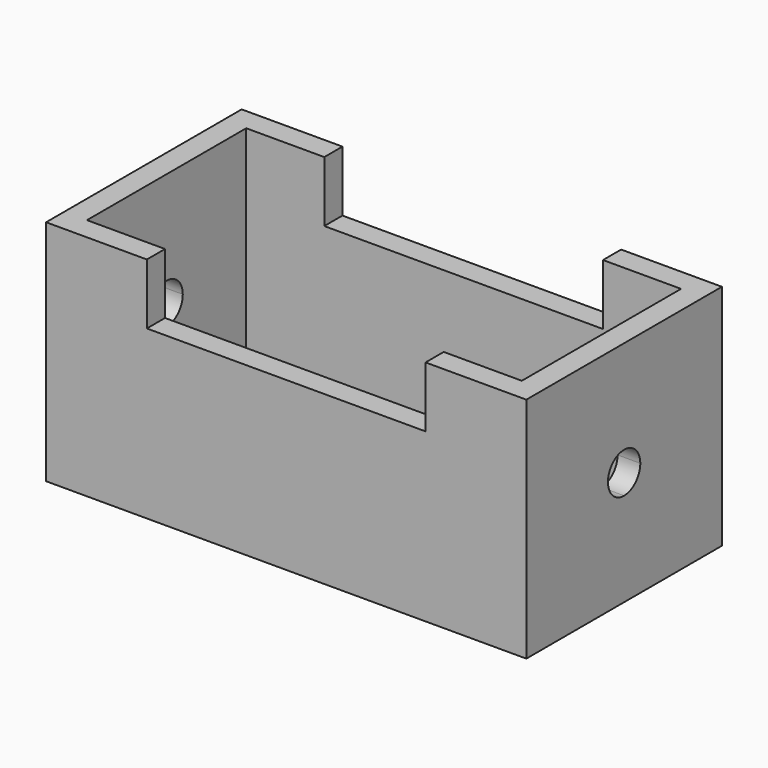
from build123d import *
from build123d import SkipClean  # not in build123d's __all__

# Parameters (mm, degrees)
F1_DEPTH = 50.8
F2_W     = 31.0465274379
F2_H     = 13.5299048007
F3_DEPTH = 25.4
F5_DEPTH = 25.4


with BuildPart() as f1:
    # F0 (on Top) → F1 (new body)
    with BuildSketch(Plane.XY):
        Polygon((-62.0559491217, 14.3422799075), (-67.1168267727, 14.3422799075), (-67.1168267727, -12.8931785002), (-13.6161604896, -12.8931785002), (-13.6161604896, -7.8323045745), (-62.0559491217, -7.8323045745), align=None)
    extrude(amount=F1_DEPTH)

    # F2 (on face) → F3 (cut)
    with BuildSketch(Plane.XZ.offset(12.8931785002)):
        with Locations((-29.1394242086, 44.0350475997)):
            Rectangle(F2_W, F2_H)
    extrude(amount=-F3_DEPTH, mode=Mode.SUBTRACT)

    # F4 (on face) → F5 (cut)
    with BuildSketch(Plane(origin=(-67.1168267727, 0, 0), x_dir=(0, -1, 0), z_dir=(-1, 0, 0))):
        with BuildLine():
            ThreePointArc((-14.3422799075, 20.8923586581), (-11.1548961475, 22.21261624), (-9.8346385657, 25.4))
            ThreePointArc((-9.8346385657, 25.4), (-11.1548961475, 28.58738376), (-14.3422799075, 29.9076413419))
            Line((-14.3422799075, 29.9076413419), (-14.3422799075, 20.8923586581))
        make_face()
    extrude(amount=-F5_DEPTH, mode=Mode.SUBTRACT)

    # F6: F1 across face


with BuildPart() as f1_1:
    add(f1.part, clean=False)
    with SkipClean():  # cleaning this boolean's faces spoils the solid; the shape is the same uncleaned
        add(f1.part.mirror(Plane(origin=(-64.5863879472, 14.3422799075, 10.4461793291), x_dir=(-1, 0, 0), z_dir=(0, 1, 0))), clean=False)

    # F7: F1 across face


with BuildPart() as f1_2:
    add(f1_1.part, clean=False)
    add(f1_1.part.mirror(Plane(origin=(-13.6161604896, 39.0473013524, 18.6350475997), x_dir=(0, 1, 0), z_dir=(1, 0, 0))), clean=False)


solid = f1_2.part
